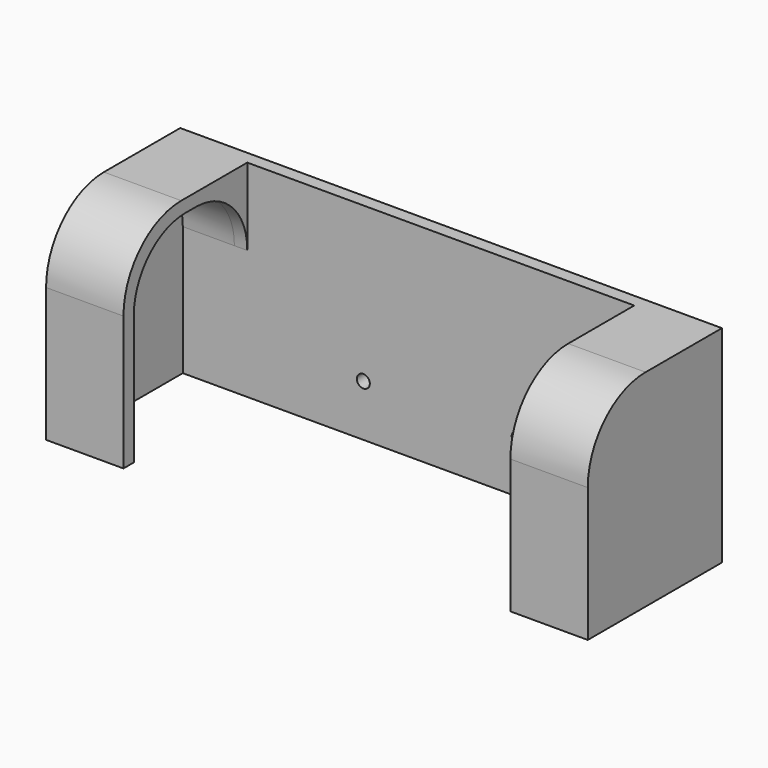
from build123d import *

# Parameters (mm, degrees)
F0_W        = 133.35
F0_H        = 50.8
F1_DEPTH    = 3.175
F2_W        = 19.05
F2_H        = 50.8
F3_DEPTH    = 38.1
F4_T        = 3.175
F4_T3_DEPTH = 57.15
F5_R        = 15.875
F7_DEPTH    = 25.4
F8_DEPTH    = 25.4
F9_R        = 1.5875
F10_DEPTH   = 25.4
F11_R       = 17.78


# Not quite as in the source:
# - a shell that OpenCascade refuses in one call is made with other operations: the cavity is built on its own and cut out


with BuildPart() as f1:
    # F0 (on Front) → F1 (new body)
    with BuildSketch(Plane.XZ):
        with Locations((66.675, 25.4)):
            Rectangle(F0_W, F0_H)
    extrude(amount=F1_DEPTH)

    # F2 (on face) → F3 (join)
    with BuildSketch(Plane.XZ.offset(3.175)):
        with Locations((9.525, 25.4)):
            Rectangle(F2_W, F2_H)
        with Locations((123.825, 25.4)):
            Rectangle(F2_W, F2_H)
    extrude(amount=F3_DEPTH)

    # F4: shell of thickness 3.175, made by hand


with BuildPart() as f4_core1:
    # F4_t2: copy of F1
    add(f1.part)

    # the walls: a layer under each face that stays
    f4_faces = [f4_core1.faces().sort_by_distance(p)[0] for p in [
        (0, -20.6375, 25.4),
        (66.675, 0, 25.4),
        (133.35, -20.6375, 25.4),
        (123.825, -41.275, 25.4),
        (114.3, -22.225, 25.4),
        (66.675, -3.175, 25.4),
        (19.05, -22.225, 25.4),
        (9.525, -41.275, 25.4),
        (123.825, -38.3267857143, 50.8),
    ]]
    thicken(f4_faces, amount=-F4_T, mode=Mode.SUBTRACT)

    # F4_s4 → F4_t3 (cut)
    with BuildSketch(Plane.XY.offset(-3.175)):
        Polygon((114.26825, -3.20675), (117.475, -3.175), (117.475, 0), (114.3, 0), align=None)
        Polygon((19.08175, -3.20675), (19.05, 0), (15.875, 0), (15.875, -3.175), align=None)
    extrude(amount=F4_T3_DEPTH, mode=Mode.SUBTRACT)


with BuildPart() as f1_1:
    add(f1.part)

    # what is left inside the walls is the cavity
    f4_cavity = [f4_core1.part.solids().sort_by_distance(p)[0] for p in [
        (3.20675, -26.458333, 23.8125),
        (130.14325, -26.458333, 23.8125),
    ]]
    add(f4_cavity, mode=Mode.SUBTRACT)

    # F5
    f5_edges = [f1_1.edges().sort_by_distance(p)[0] for p in [
        (9.525, -3.175, 47.625),
        (123.825, -3.175, 47.625),
        (9.525, -38.1, 47.625),
        (123.825, -38.1, 47.625),
    ]]
    fillet(f5_edges, radius=F5_R)

    # F6 (on face) → F7 (cut)
    with BuildSketch(Plane(origin=(15.875, 0, 0), x_dir=(0, -1, 0), z_dir=(-1, 0, 0))):
        with BuildLine():
            ThreePointArc((19.05, 47.625), (7.8246798487, 42.9753201513), (3.175, 31.75))
            Line((3.175, 31.75), (3.175, 0))
            Line((3.175, 0), (38.1, 0))
            Line((38.1, 0), (38.1, 31.75))
            ThreePointArc((38.1, 31.75), (33.4503201513, 42.9753201513), (22.225, 47.625))
            Line((22.225, 47.625), (19.05, 47.625))
        make_face()
    extrude(amount=-F7_DEPTH, mode=Mode.SUBTRACT)

    # F8 (cut): a face of the model
    f8_faces = [f1_1.faces().sort_by_distance(p)[0] for p in [
        (117.475, -20.6375, 22.4028811498),
    ]]
    extrude(f8_faces, amount=-F8_DEPTH, mode=Mode.SUBTRACT)

    # F9 (on face) → F10 (cut)
    with BuildSketch(Plane(origin=(0, 0, 0), x_dir=(-1, 0, 0), z_dir=(0, 1, 0))):
        with Locations((-47.625, 12.7)):
            Circle(F9_R)
        with Locations((-85.725, 12.7)):
            Circle(F9_R)
    extrude(amount=-F10_DEPTH, mode=Mode.SUBTRACT)

    # F11
    f11_edges = [f1_1.edges().sort_by_distance(p)[0] for p in [
        (9.525, -41.275, 50.8),
        (123.825, -41.275, 50.8),
    ]]
    fillet(f11_edges, radius=F11_R)


solid = f1_1.part
